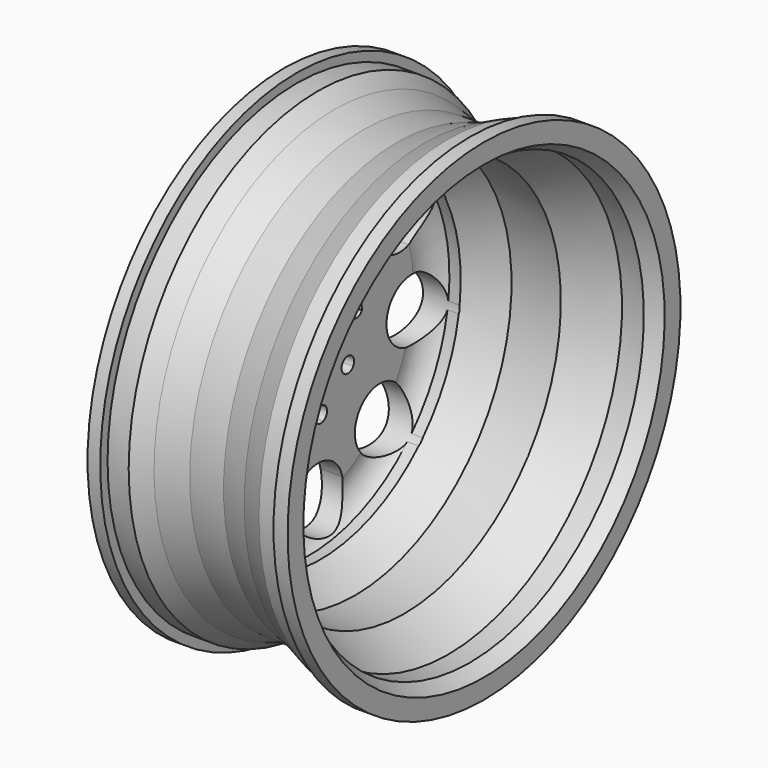
from build123d import *

# Parameters (mm, degrees)
F2_R     = 17.4118319202
F3_DEPTH = 50
F4_DEPTH = 30
F5_DEPTH = 50


# Not quite as in the source:
# - a feature names something its author has since deleted; it is built from what else it names


with BuildPart() as f1:
    # F0 (on Front) → F1 (revolve)
    with BuildSketch(Plane.XZ):
        with BuildLine():
            Line((-25.5366545171, 46.2463870645), (-25.5366545171, 0))
            Line((-25.5366545171, 0), (-18.5301266611, 0))
            Line((-18.5301266611, 0), (-18.5301266611, 46.4724041522))
            ThreePointArc((-18.5301266611, 46.4724041522), (-18.0433446656, 51.8988411255), (-14.6878389642, 56.1911314726))
            Line((-14.6878389642, 56.1911314726), (-11.0715664923, 56.1911314726))
            Line((-11.0715664923, 56.1911314726), (0, 62.7456232905))
            Line((0, 62.7456232905), (3.845551284, 62.7456232905))
            Line((3.845551284, 62.7456232905), (15.8244501799, 62.7456232905))
            Line((15.8244501799, 62.7456232905), (29.837500304, 69.7521492839))
            Line((29.837500304, 69.7521492839), (36.8440262973, 69.7521492839))
            Line((36.8440262973, 69.7521492839), (41.364364326, 72.4643543363))
            Line((41.364364326, 72.4643543363), (41.364364326, 78.7928253412))
            Line((41.364364326, 78.7928253412), (36.8440262973, 78.7928253412))
            Line((36.8440262973, 78.7928253412), (36.8440262973, 75.8546069264))
            Line((36.8440262973, 75.8546069264), (29.837500304, 75.8546069264))
            Line((29.837500304, 75.8546069264), (22.3789419979, 72.4643543363))
            Line((22.3789419979, 72.4643543363), (13.5642802343, 69.7521492839))
            Line((13.5642802343, 69.7521492839), (2.715466544, 69.7521492839))
            Line((2.715466544, 69.7521492839), (-6.5512284636, 72.4643543363))
            Line((-6.5512284636, 72.4643543363), (-11.9756357744, 75.8546069264))
            Line((-11.9756357744, 75.8546069264), (-18.7561437488, 75.8546069264))
            Line((-18.7561437488, 75.8546069264), (-18.7561437488, 78.7928253412))
            Line((-18.7561437488, 78.7928253412), (-22.8244494647, 78.7928253412))
            Line((-22.8244494647, 78.7928253412), (-22.8244494647, 72.4643543363))
            Line((-22.8244494647, 72.4643543363), (-16.043940559, 69.7521492839))
            Line((-16.043940559, 69.7521492839), (-11.9756357744, 69.7521492839))
            Line((-11.9756357744, 69.7521492839), (-6.5512284636, 65.6838417053))
            Line((-6.5512284636, 65.6838417053), (-12.2016528621, 62.9716441035))
            Line((-12.2016528621, 62.9716441035), (-16.043940559, 62.9716441035))
            ThreePointArc((-16.043940559, 62.9716441035), (-22.9980693093, 55.8620753044), (-25.5366545171, 46.2463870645))
        make_face()
    revolve(axis=Axis((-22.0333905891, 0, 0), (-1, 0, 0)))

    # F2 (on face) → F3 (cut)
    with BuildSketch(Plane(origin=(-25.5366545171, 0, 0), x_dir=(0, -1, 0), z_dir=(-1, 0, 0))):
        Circle(F2_R)
    extrude(amount=-F3_DEPTH, mode=Mode.SUBTRACT)

    # F2 (on face) → F4 (cut)
    with BuildSketch(Plane(origin=(-25.5366545171, 0, 0), x_dir=(0, -1, 0), z_dir=(-1, 0, 0))):
        with BuildLine():
            ThreePointArc((-28.9641792858, 36.0528034252), (-17.7326916391, 31.8374870451), (-10.536931292, 41.4362494638))
            ThreePointArc((-10.536931292, 41.4362494638), (-10.6912499296, 43.1862661808), (-11.149442994, 44.8822708588))
            ThreePointArc((-11.149442994, 44.8822708588), (-20.536931292, 41.4362494638), (-28.9641792858, 36.0528034252))
        make_face()
        with BuildLine():
            ThreePointArc((-28.9641792858, 36.0528034252), (-20.536931292, 41.4362494638), (-11.149442994, 44.8822708588))
            ThreePointArc((-11.149442994, 44.8822708588), (-24.9776957702, 50.3961384614), (-28.9641792858, 36.0528034252))
        make_face()
        with BuildLine():
            ThreePointArc((17.3610480402, 42.863998034), (7.7408899176, 45.5939353401), (-2.2412071132, 46.1920480948))
            ThreePointArc((-2.2412071132, 46.1920480948), (6.0670532335, 35.7350170042), (17.3610480402, 42.863998034))
        make_face()
        with BuildLine():
            ThreePointArc((17.7408899176, 45.5939353401), (8.0400802348, 55.5894585958), (-2.2412071132, 46.1920480948))
            ThreePointArc((-2.2412071132, 46.1920480948), (7.7408899176, 45.5939353401), (17.3610480402, 42.863998034))
            ThreePointArc((17.3610480402, 42.863998034), (17.6454742407, 44.2158172803), (17.7408899176, 45.5939353401))
        make_face()
        with BuildLine():
            ThreePointArc((39.2402088034, 24.473134854), (33.0619542818, 32.3362875974), (25.3378300008, 38.6875004022))
            ThreePointArc((25.3378300008, 38.6875004022), (25.9128651571, 25.3441116351), (39.2402088034, 24.473134854))
        make_face()
        with BuildLine():
            ThreePointArc((43.0619542818, 32.3362875974), (36.4352877362, 41.7501402309), (25.3378300008, 38.6875004022))
            ThreePointArc((25.3378300008, 38.6875004022), (33.0619542818, 32.3362875974), (39.2402088034, 24.473134854))
            ThreePointArc((39.2402088034, 24.473134854), (42.0559118427, 27.9649345584), (43.0619542818, 32.3362875974))
        make_face()
        with BuildLine():
            ThreePointArc((46.2220130859, 1.5012737277), (44.8075206553, 11.4461525957), (41.2790889585, 20.8510223077))
            ThreePointArc((41.2790889585, 20.8510223077), (33.5411063309, 8.5681290926), (46.2220130859, 1.5012737277))
        make_face()
        with BuildLine():
            ThreePointArc((53.2299757755, 11.0431662409), (49.5739150813, 18.7732654696), (41.2790889585, 20.8510223077))
            ThreePointArc((41.2790889585, 20.8510223077), (44.8075206553, 11.4461525957), (46.2220130859, 1.5012737277))
            ThreePointArc((46.2220130859, 1.5012737277), (51.2897640204, 5.1237225636), (53.2299757755, 11.0431662409))
        make_face()
        with BuildLine():
            ThreePointArc((35.4012257601, -29.7570417077), (40.9703427727, -21.4513246586), (44.6238194275, -12.1426132369))
            ThreePointArc((44.6238194275, -12.1426132369), (32.1111982268, -16.812838061), (35.4012257601, -29.7570417077))
        make_face()
        with BuildLine():
            ThreePointArc((50.9703427727, -21.4513246586), (49.2327506102, -15.8181535511), (44.6238194275, -12.1426132369))
            ThreePointArc((44.6238194275, -12.1426132369), (40.9703427727, -21.4513246586), (35.4012257601, -29.7570417077))
            ThreePointArc((35.4012257601, -29.7570417077), (45.6771904372, -30.2743391696), (50.9703427727, -21.4513246586))
        make_face()
        with BuildLine():
            ThreePointArc((28.9641792858, -36.0528034252), (20.536931292, -41.4362494638), (11.149442994, -44.8822708588))
            ThreePointArc((11.149442994, -44.8822708588), (22.2869480091, -51.2819308262), (30.536931292, -41.4362494638))
            ThreePointArc((30.536931292, -41.4362494638), (30.1356937106, -38.6320098109), (28.9641792858, -36.0528034252))
        make_face()
        with BuildLine():
            ThreePointArc((28.9641792858, -36.0528034252), (16.0961668138, -32.4763604662), (11.149442994, -44.8822708588))
            ThreePointArc((11.149442994, -44.8822708588), (20.536931292, -41.4362494638), (28.9641792858, -36.0528034252))
        make_face()
        with BuildLine():
            ThreePointArc((1.5960199926, -46.2188385477), (-8.4290299561, -45.4717469481), (-18.0557890878, -42.5760119895))
            ThreePointArc((-18.0557890878, -42.5760119895), (-10.11925265, -54.5899229453), (1.5960199926, -46.2188385477))
        make_face()
        with BuildLine():
            ThreePointArc((1.7033826932, -44.7574257851), (-7.1992836772, -34.8178151838), (-18.0557890878, -42.5760119895))
            ThreePointArc((-18.0557890878, -42.5760119895), (-8.4290299561, -45.4717469481), (1.5960199926, -46.2188385477))
            ThreePointArc((1.5960199926, -46.2188385477), (1.6765059, -45.4901013634), (1.7033826932, -44.7574257851))
        make_face()
        with BuildLine():
            ThreePointArc((-25.3378300008, -38.6875004022), (-33.0619542818, -32.3362875974), (-39.2402088034, -24.473134854))
            ThreePointArc((-39.2402088034, -24.473134854), (-40.2110434065, -39.3284635597), (-25.3378300008, -38.6875004022))
        make_face()
        with BuildLine():
            ThreePointArc((-23.0619542818, -32.3362875974), (-28.6906012427, -23.3423300365), (-39.2402088034, -24.473134854))
            ThreePointArc((-39.2402088034, -24.473134854), (-33.0619542818, -32.3362875974), (-25.3378300008, -38.6875004022))
            ThreePointArc((-25.3378300008, -38.6875004022), (-23.6481016483, -35.7096210519), (-23.0619542818, -32.3362875974))
        make_face()
        with BuildLine():
            ThreePointArc((-43.2386772557, -16.4056424957), (-45.7544758449, -6.7272770625), (-46.1309435293, 3.265634029))
            ThreePointArc((-46.1309435293, 3.265634029), (-55.6481083531, -8.1819370888), (-43.2386772557, -16.4056424957))
        make_face()
        with BuildLine():
            ThreePointArc((-35.7544758449, -6.7272770625), (-38.817786319, 0.4756625056), (-46.1309435293, 3.265634029))
            ThreePointArc((-46.1309435293, 3.265634029), (-45.7544758449, -6.7272770625), (-43.2386772557, -16.4056424957))
            ThreePointArc((-43.2386772557, -16.4056424957), (-37.8437873195, -12.8445482723), (-35.7544758449, -6.7272770625))
        make_face()
        with BuildLine():
            ThreePointArc((-44.6238194275, 12.1426132369), (-40.9703427727, 21.4513246586), (-35.4012257601, 29.7570417077))
            ThreePointArc((-35.4012257601, 29.7570417077), (-49.8294873185, 26.0898112562), (-44.6238194275, 12.1426132369))
        make_face()
        with BuildLine():
            ThreePointArc((-30.9703427727, 21.4513246586), (-32.1473282616, 26.1581723231), (-35.4012257601, 29.7570417077))
            ThreePointArc((-35.4012257601, 29.7570417077), (-40.9703427727, 21.4513246586), (-44.6238194275, 12.1426132369))
            ThreePointArc((-44.6238194275, 12.1426132369), (-35.3371716652, 13.188916821), (-30.9703427727, 21.4513246586))
        make_face()
    extrude(amount=-F4_DEPTH, mode=Mode.SUBTRACT)

    # F2 (on face) → F5 (cut)
    with BuildSketch(Plane(origin=(-25.5366545171, 0, 0), x_dir=(0, -1, 0), z_dir=(-1, 0, 0))):
        with BuildLine():
            ThreePointArc((-2.5037225274, 22.9016763906), (-3.4359333957, 24.8489917833), (-5.5373523183, 25.3440603175))
            ThreePointArc((-5.5373523183, 25.3440603175), (-6.571511659, 20.9543609979), (-2.5037225274, 22.9016763906))
        make_face()
        with BuildLine():
            ThreePointArc((11.9131710754, 21.4689597079), (11.5059807252, 22.8364931699), (10.4170528595, 23.7585494885))
            ThreePointArc((10.4170528595, 23.7585494885), (7.3203614256, 20.1014262458), (11.9131710754, 21.4689597079))
        make_face()
        with BuildLine():
            ThreePointArc((22.7345532693, 11.8358301198), (22.6475246398, 12.4897178512), (22.392497937, 13.0980800202))
            ThreePointArc((22.392497937, 13.0980800202), (17.8215818988, 11.1819423883), (22.7345532693, 11.8358301198))
        make_face()
        with BuildLine():
            ThreePointArc((25.8270238615, -2.318184289), (20.8300892936, -2.1944193367), (25.8147696508, -2.5654106792))
            ThreePointArc((25.8147696508, -2.5654106792), (25.8239584294, -2.4419492413), (25.8270238615, -2.318184289))
        make_face()
        with BuildLine():
            ThreePointArc((20.009364195, -15.5867310915), (15.1728837216, -14.6974285571), (19.3766769968, -17.2490014968))
            ThreePointArc((19.3766769968, -17.2490014968), (19.8458446683, -16.4760336259), (20.009364195, -15.5867310915))
        make_face()
        with BuildLine():
            ThreePointArc((7.5037225274, -22.9016763906), (3.0564071361, -21.3338872572), (5.537352314, -25.3440603185))
            ThreePointArc((5.537352314, -25.3440603185), (6.9510379187, -24.469465524), (7.5037225274, -22.9016763906))
        make_face()
        with BuildLine():
            ThreePointArc((-17.7345532693, -11.8358301198), (-20.8884411947, -9.4228588019), (-22.3924977341, -13.098080367))
            ThreePointArc((-22.3924977341, -13.098080367), (-19.5806653439, -14.2488014377), (-17.7345532693, -11.8358301198))
        make_face()
        with BuildLine():
            ThreePointArc((-21.2213149667, 2.4514952675), (-22.8538313364, 4.7961641463), (-25.6192926877, 4.078664764))
            ThreePointArc((-25.6192926877, 4.078664764), (-25.8044944397, 2.6667828528), (-25.9119468497, 1.2468658834))
            ThreePointArc((-25.9119468497, 1.2468658834), (-23.0994547363, 0.0300721624), (-21.2213149667, 2.4514952675))
        make_face()
        with BuildLine():
            ThreePointArc((-15.009364195, 15.5867310915), (-16.6200616606, 17.9232115649), (-19.3766769968, 17.2490014968))
            ThreePointArc((-19.3766769968, 17.2490014968), (-18.3986667294, 13.2502506182), (-15.009364195, 15.5867310915))
        make_face()
        with BuildLine():
            ThreePointArc((-6.9131710754, -21.4689597079), (-10.7807045685, -19.3761500783), (-10.4170527917, -23.7585495182))
            ThreePointArc((-10.4170527917, -23.7585495182), (-8.0456375824, -23.5617693374), (-6.9131710754, -21.4689597079))
        make_face()
    extrude(amount=-F5_DEPTH, mode=Mode.SUBTRACT)


solid = f1.part
